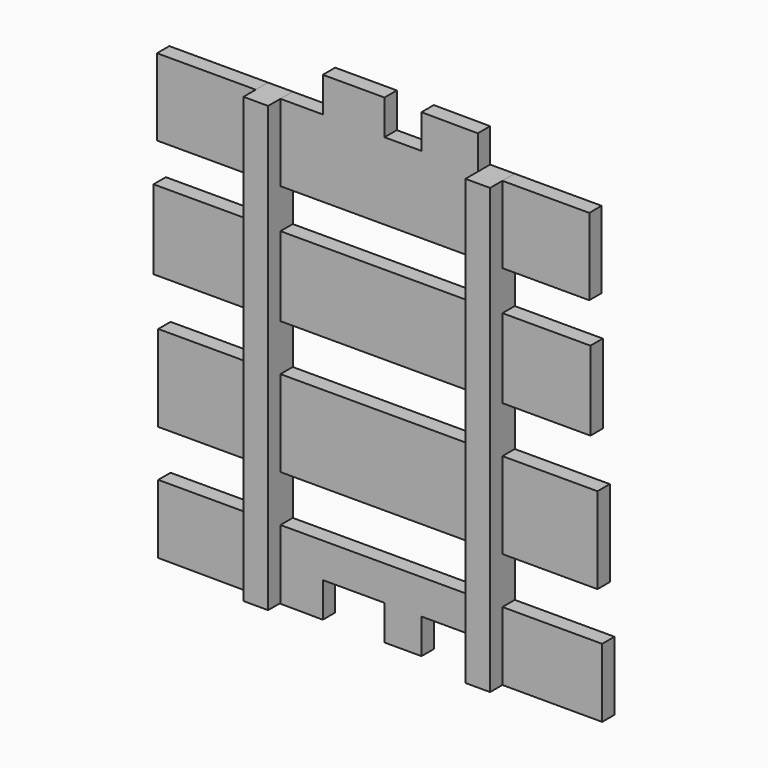
from build123d import *

# Parameters (mm, degrees)
F0_W     = 12.7
F0_H     = 7.1991272271
F1_DEPTH = 3.175
F0_W_2   = 40.64
F0_H_2   = 16.3149703294
F0_H_3   = 17.7578479052
F0_W_3   = 20.0888210887
F0_W_4   = 21.0607587677
F0_W_5   = 20.3408464175
F0_H_4   = 15.8380791545
F0_W_6   = 17.8883576828
F0_W_7   = 18.128329708
F0_W_8   = 19.5802114373
F0_W_9   = 5.08
F0_H_5   = 8.1590097398
F0_H_6   = 9.6018854529
F0_H_7   = 9.5988344401
F0_H_8   = 14.158282429
F2_DEPTH = 6.35


# Not quite as in the source:
# - a feature names something its author has since deleted; it is built from what else it names


with BuildPart() as f1:
    # F0 (on Front) → F1 (new body)
    with BuildSketch(Plane.XZ):
        Polygon((-14.6131411788, 40.3120592237), (-23.3456920832, 40.3120592237), (-23.3456920832, 24.4739800692), (17.2943079168, 24.4739800692), (17.2943079168, 40.3120592237), (5.7068588212, 40.3120592237), (-1.9131411788, 40.3120592237), align=None)
        with Locations((-8.2631411788, 43.9116228372)):
            Rectangle(F0_W, F0_H)
        Polygon((5.7068588212, 40.3120592237), (17.2943079168, 40.3120592237), (17.2943079168, 47.2727881546), (5.7068588212, 47.3364423823), align=None)
    extrude(amount=F1_DEPTH)


with BuildPart() as f1b:
    # F0 (on Front) → F1, piece 2 (new body)
    with BuildSketch(Plane.XZ):
        with Locations((-3.0256920832, 8.1574851647)):
            Rectangle(F0_W_2, F0_H_2)
    extrude(amount=F1_DEPTH)


with BuildPart() as f1c:
    # F0 (on Front) → F1, piece 3 (new body)
    with BuildSketch(Plane.XZ):
        with Locations((-3.0256920832, -18.4808094054)):
            Rectangle(F0_W_2, F0_H_3)
    extrude(amount=F1_DEPTH)


with BuildPart() as f1d:
    # F0 (on Front) → F1, piece 4 (new body)
    with BuildSketch(Plane.XZ):
        Polygon((-28.4256920832, -51.1168502271), (-28.4256920832, -36.9585677981), (-48.5145131719, -36.9585677981), (-48.5145131719, -51.1168502271), (-14.6131411788, -51.296133548), (-14.6131411788, -44.107933548), (-1.9131411788, -44.107933548), (-1.9131411788, -51.296133548), (5.7068588212, -51.296133548), (5.7068588212, -44.107933548), (17.2943079168, -44.107933548), (17.2943079168, -36.9585677981), (-23.3456920832, -36.9585677981), (-23.3456920832, -51.1168502271), align=None)
    extrude(amount=F1_DEPTH)


with BuildPart() as f1e:
    # F0 (on Front) → F1, piece 5 (new body)
    with BuildSketch(Plane.XZ):
        with Locations((-38.4701026276, -18.4808094054)):
            Rectangle(F0_W_3, F0_H_3)
    extrude(amount=F1_DEPTH)


with BuildPart() as f1f:
    # F0 (on Front) → F1, piece 6 (new body)
    with BuildSketch(Plane.XZ):
        with Locations((-38.9560714671, 8.1574851647)):
            Rectangle(F0_W_4, F0_H_2)
    extrude(amount=F1_DEPTH)


with BuildPart() as f1g:
    # F0 (on Front) → F1, piece 7 (new body)
    with BuildSketch(Plane.XZ):
        with Locations((-38.596115292, 32.3930196464)):
            Rectangle(F0_W_5, F0_H_4)
    extrude(amount=F1_DEPTH)


with BuildPart() as f1h:
    # F0 (on Front) → F1, piece 8 (new body)
    with BuildSketch(Plane.XZ):
        with Locations((31.3184867582, 32.3930196464)):
            Rectangle(F0_W_6, F0_H_4)
    extrude(amount=F1_DEPTH)


with BuildPart() as f1i:
    # F0 (on Front) → F1, piece 9 (new body)
    with BuildSketch(Plane.XZ):
        with Locations((31.4384727708, 8.1574851647)):
            Rectangle(F0_W_7, F0_H_2)
    extrude(amount=F1_DEPTH)


with BuildPart() as f1j:
    # F0 (on Front) → F1, piece 10 (new body)
    with BuildSketch(Plane.XZ):
        with Locations((32.1644136354, -18.4808094054)):
            Rectangle(F0_W_8, F0_H_3)
    extrude(amount=F1_DEPTH)


with BuildPart() as f1k:
    # F0 (on Front) → F1, piece 11 (new body)
    with BuildSketch(Plane.XZ):
        Polygon((42.9144074547, -36.9585677981), (22.3743079168, -36.9585677981), (22.3743079168, -51.1001323521), (42.9144074547, -51.1168502271), align=None)
    extrude(amount=F1_DEPTH)


with BuildPart() as f2:
    # F0 (on Front) → F2 (new body)
    with BuildSketch(Plane.XZ):
        with Locations((-25.8856920832, 20.3944751993)):
            Rectangle(F0_W_9, F0_H_5)
        with Locations((-25.8856920832, 32.3930196464)):
            Rectangle(F0_W_9, F0_H_4)
        with Locations((-25.8856920832, 8.1574851647)):
            Rectangle(F0_W_9, F0_H_2)
        with Locations((-25.8856920832, -4.8009427264)):
            Rectangle(F0_W_9, F0_H_6)
        with Locations((-25.8856920832, -18.4808094054)):
            Rectangle(F0_W_9, F0_H_3)
        with Locations((-25.8856920832, -32.1591505781)):
            Rectangle(F0_W_9, F0_H_7)
        with Locations((-25.8856920832, -44.0377090126)):
            Rectangle(F0_W_9, F0_H_8)
    extrude(amount=F2_DEPTH)


with BuildPart() as f2b:
    # F0 (on Front) → F2, piece 2 (new body)
    with BuildSketch(Plane.XZ):
        Polygon((22.3743079168, -36.9585677981), (17.2943079168, -36.9585677981), (17.2943079168, -44.107933548), (17.2943079168, -51.1001323521), (22.3743079168, -51.1001323521), align=None)
        with Locations((19.8343079168, -32.1591505781)):
            Rectangle(F0_W_9, F0_H_7)
        with Locations((19.8343079168, -18.4808094054)):
            Rectangle(F0_W_9, F0_H_3)
        with Locations((19.8343079168, -4.8009427264)):
            Rectangle(F0_W_9, F0_H_6)
        with Locations((19.8343079168, 8.1574851647)):
            Rectangle(F0_W_9, F0_H_2)
        with Locations((19.8343079168, 20.3944751993)):
            Rectangle(F0_W_9, F0_H_5)
        with Locations((19.8343079168, 32.3930196464)):
            Rectangle(F0_W_9, F0_H_4)
    extrude(amount=F2_DEPTH)


solid = Compound([f1.part, f1b.part, f1c.part, f1d.part, f1e.part, f1f.part, f1g.part, f1h.part, f1i.part, f1j.part, f1k.part, f2.part, f2b.part])
